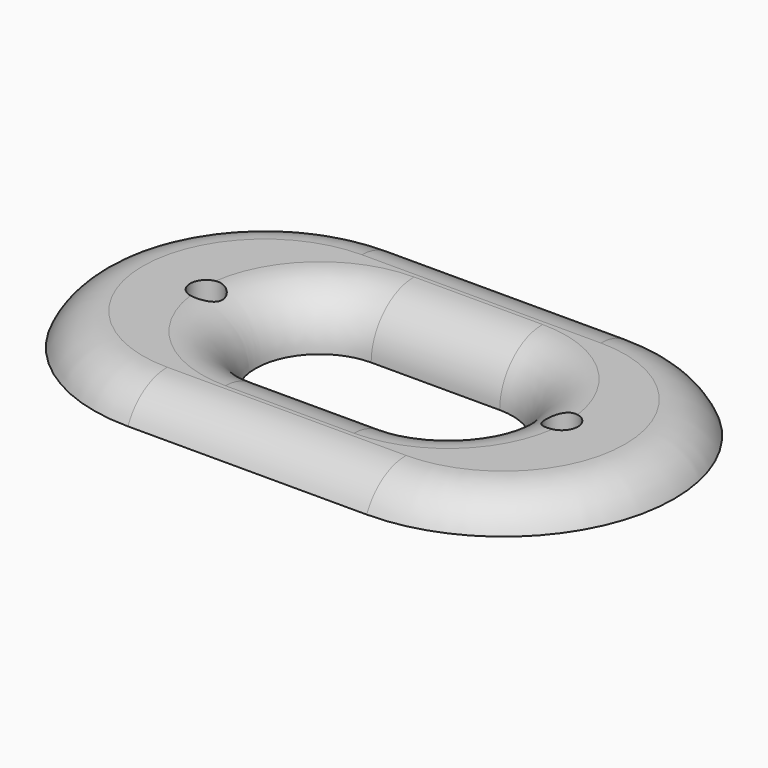
from build123d import *

# Parameters (mm, degrees)
F0_R        = 1.5
F1_DEPTH    = 2
F2_DEPTH    = 3
F3_T1_DEPTH = 12
F3_T4_ANGLE = 180
F3_T6_ANGLE = 180
F4_T1_DEPTH = 22.3
F4_T4_ANGLE = 180
F4_T6_ANGLE = 180


# Not quite as in the source:
# - a fillet or chamfer that OpenCascade refuses, or shapes differently, is made with other operations: its cross-section is extruded or revolved along the edge and cut away or added


with BuildPart() as f1:
    # F0 (on Top) → F1 (new body)
    with BuildSketch(Plane.XY):
        with BuildLine():
            Line((-11.15, -7.95), (11.15, -7.95))
            ThreePointArc((11.15, -7.95), (19.1, 0), (11.15, 7.95))
            Line((11.15, 7.95), (-11.15, 7.95))
            ThreePointArc((-11.15, 7.95), (-19.1, 0), (-11.15, -7.95))
        make_face()
        with Locations((-16.6, 0)):
            Circle(F0_R, mode=Mode.SUBTRACT)
        with BuildLine():
            Line((-6, 6), (6, 6))
            ThreePointArc((6, 6), (10.2426406871, 4.2426406871), (12, 0))
            ThreePointArc((12, 0), (10.2426406871, -4.2426406871), (6, -6))
            Line((6, -6), (-6, -6))
            ThreePointArc((-6, -6), (-12, 0), (-6, 6))
        make_face(mode=Mode.SUBTRACT)
        with Locations((16.6, 0)):
            Circle(F0_R, mode=Mode.SUBTRACT)
    extrude(amount=-F1_DEPTH)

    # F0 (on Top) → F2 (join)
    with BuildSketch(Plane.XY):
        with BuildLine():
            Line((11.15, 15.95), (-11.15, 15.95))
            ThreePointArc((-11.15, 15.95), (-27.1, 0), (-11.15, -15.95))
            Line((-11.15, -15.95), (11.15, -15.95))
            ThreePointArc((11.15, -15.95), (27.1, 0), (11.15, 15.95))
        make_face()
        with BuildLine():
            ThreePointArc((11.15, 7.95), (19.1, 0), (11.15, -7.95))
            Line((11.15, -7.95), (-11.15, -7.95))
            ThreePointArc((-11.15, -7.95), (-19.1, 0), (-11.15, 7.95))
            Line((-11.15, 7.95), (11.15, 7.95))
        make_face(mode=Mode.SUBTRACT)
        with BuildLine():
            Line((-11.15, -7.95), (11.15, -7.95))
            ThreePointArc((11.15, -7.95), (19.1, 0), (11.15, 7.95))
            Line((11.15, 7.95), (-11.15, 7.95))
            ThreePointArc((-11.15, 7.95), (-19.1, 0), (-11.15, -7.95))
        make_face()
        with Locations((-16.6, 0)):
            Circle(F0_R, mode=Mode.SUBTRACT)
        with BuildLine():
            Line((-6, 6), (6, 6))
            ThreePointArc((6, 6), (10.2426406871, 4.2426406871), (12, 0))
            ThreePointArc((12, 0), (10.2426406871, -4.2426406871), (6, -6))
            Line((6, -6), (-6, -6))
            ThreePointArc((-6, -6), (-12, 0), (-6, 6))
        make_face(mode=Mode.SUBTRACT)
        with Locations((16.6, 0)):
            Circle(F0_R, mode=Mode.SUBTRACT)
    extrude(amount=F2_DEPTH)

    # F3: fillet of radius 5 on 4 edges, made by hand

    # F3_s2 → F3_t1 (cut)
    with BuildSketch(Plane.YZ.offset(-6)):
        with BuildLine():
            ThreePointArc((11, 3), (7.4644660941, 1.5355339059), (6, -2))
            Line((6, -2), (6, 3))
            Line((6, 3), (11, 3))
        make_face()
        with BuildLine():
            ThreePointArc((-11, 3), (-7.4644660941, 1.5355339059), (-6, -2))
            Line((-6, -2), (-6, 3))
            Line((-6, 3), (-11, 3))
        make_face()
    extrude(amount=F3_T1_DEPTH, mode=Mode.SUBTRACT)

    # F3_s3 → F3_t4 (revolve, cut)
    with BuildSketch(Plane.YZ.offset(-6)):
        with BuildLine():
            ThreePointArc((-11, 3), (-7.4644660941, 1.5355339059), (-6, -2))
            Line((-6, -2), (-6, 3))
            Line((-6, 3), (-11, 3))
        make_face()
    revolve(axis=Axis((-6, 0, 3), (0, 0, -1)), revolution_arc=F3_T4_ANGLE, mode=Mode.SUBTRACT)

    # F3_s5 → F3_t6 (revolve, cut)
    with BuildSketch(Plane.YZ.offset(6)):
        with BuildLine():
            ThreePointArc((11, 3), (7.4644660941, 1.5355339059), (6, -2))
            Line((6, -2), (6, 3))
            Line((6, 3), (11, 3))
        make_face()
    revolve(axis=Axis((6, 0, 3), (0, 0, -1)), revolution_arc=F3_T6_ANGLE, mode=Mode.SUBTRACT)

    # F4: fillet of radius 5 on 1 edges, made by hand

    # F4_s2 → F4_t1 (cut)
    with BuildSketch(Plane.YZ.offset(-11.15)):
        with BuildLine():
            ThreePointArc((11.367424305, 3), (14.1060370926, 2.1833001327), (15.95, 0))
            Line((15.95, 0), (15.95, 3))
            Line((15.95, 3), (11.367424305, 3))
        make_face()
        with BuildLine():
            ThreePointArc((-11.367424305, 3), (-14.1060370926, 2.1833001327), (-15.95, 0))
            Line((-15.95, 0), (-15.95, 3))
            Line((-15.95, 3), (-11.367424305, 3))
        make_face()
    extrude(amount=F4_T1_DEPTH, mode=Mode.SUBTRACT)

    # F4_s3 → F4_t4 (revolve, cut)
    with BuildSketch(Plane.YZ.offset(11.15)):
        with BuildLine():
            ThreePointArc((-11.367424305, 3), (-14.1060370926, 2.1833001327), (-15.95, 0))
            Line((-15.95, 0), (-15.95, 3))
            Line((-15.95, 3), (-11.367424305, 3))
        make_face()
    revolve(axis=Axis((11.15, 0, 3), (0, 0, 1)), revolution_arc=F4_T4_ANGLE, mode=Mode.SUBTRACT)

    # F4_s5 → F4_t6 (revolve, cut)
    with BuildSketch(Plane.YZ.offset(-11.15)):
        with BuildLine():
            ThreePointArc((11.367424305, 3), (14.1060370926, 2.1833001327), (15.95, 0))
            Line((15.95, 0), (15.95, 3))
            Line((15.95, 3), (11.367424305, 3))
        make_face()
    revolve(axis=Axis((-11.15, 0, 3), (0, 0, 1)), revolution_arc=F4_T6_ANGLE, mode=Mode.SUBTRACT)


with BuildPart() as f5_1:
    # F5: copy of F1
    add(f1.part.moved(Location((0, 28, 23))))


solid = f1.part
